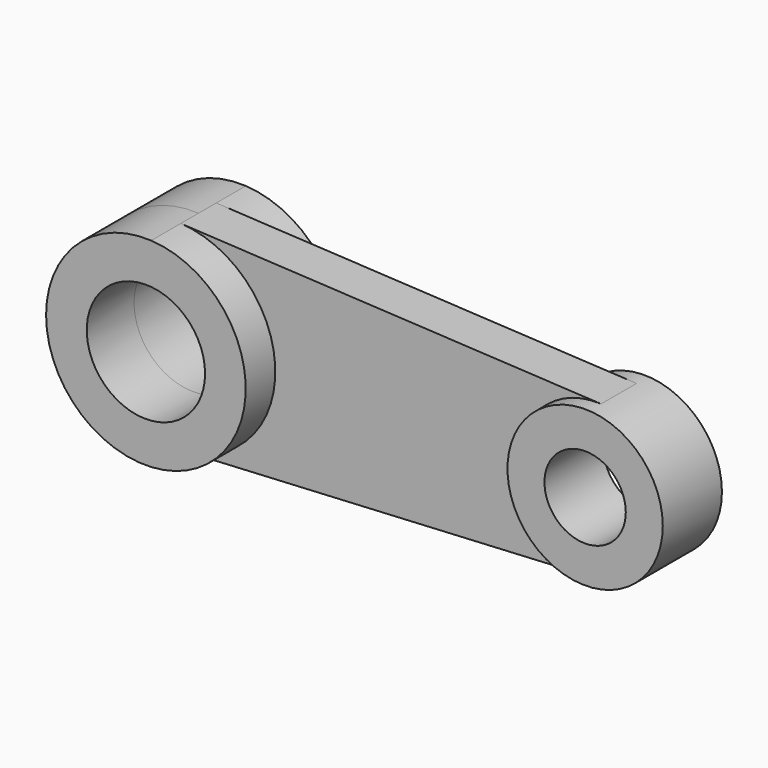
from build123d import *

# Parameters (mm, degrees)
F1_DEPTH = 9.525
F0_R     = 17.4625
F2_DEPTH = 15.875
F0_R_2   = 25.4
F3_DEPTH = 25.4


with BuildPart() as f1:
    # F0 (on Front) → F1 (new body, symmetric)
    with BuildSketch(Plane.XZ):
        with BuildLine():
            ThreePointArc((-150.9907119117, 42.803092487), (-122.150907194, 29.4999956791), (-110.3841329643, 0))
            ThreePointArc((-110.3841329643, 0), (-122.150907194, -29.4999956791), (-150.9907119117, -42.803092487))
            Line((-150.9907119117, -42.803092487), (29.4829722989, -33.2912941566))
            ThreePointArc((29.4829722989, -33.2912941566), (-5.6091329643, 0), (29.4829722989, 33.2912941566))
            Line((29.4829722989, 33.2912941566), (-150.9907119117, 42.803092487))
        make_face()
    extrude(amount=F1_DEPTH, both=True)

    # F0 (on Front) → F2 (join, symmetric)
    with BuildSketch(Plane.XZ):
        with BuildLine():
            ThreePointArc((61.0658670357, 0), (51.9139315238, 22.9444410837), (29.4829722989, 33.2912941566))
            ThreePointArc((29.4829722989, 33.2912941566), (-5.6091329643, 0), (29.4829722989, -33.2912941566))
            ThreePointArc((29.4829722989, -33.2912941566), (51.9139315238, -22.9444410837), (61.0658670357, 0))
        make_face()
        with Locations((27.7283670357, 0)):
            Circle(F0_R, mode=Mode.SUBTRACT)
    extrude(amount=F2_DEPTH, both=True)

    # F0 (on Front) → F3 (join, symmetric)
    with BuildSketch(Plane.XZ):
        with BuildLine():
            ThreePointArc((-150.9907119117, -42.803092487), (-122.150907194, -29.4999956791), (-110.3841329643, 0))
            ThreePointArc((-110.3841329643, 0), (-122.150907194, 29.4999956791), (-150.9907119117, 42.803092487))
            ThreePointArc((-150.9907119117, 42.803092487), (-196.1091329643, 0), (-150.9907119117, -42.803092487))
        make_face()
        with Locations((-153.2466329643, 0)):
            Circle(F0_R_2, mode=Mode.SUBTRACT)
    extrude(amount=F3_DEPTH, both=True)


solid = f1.part
